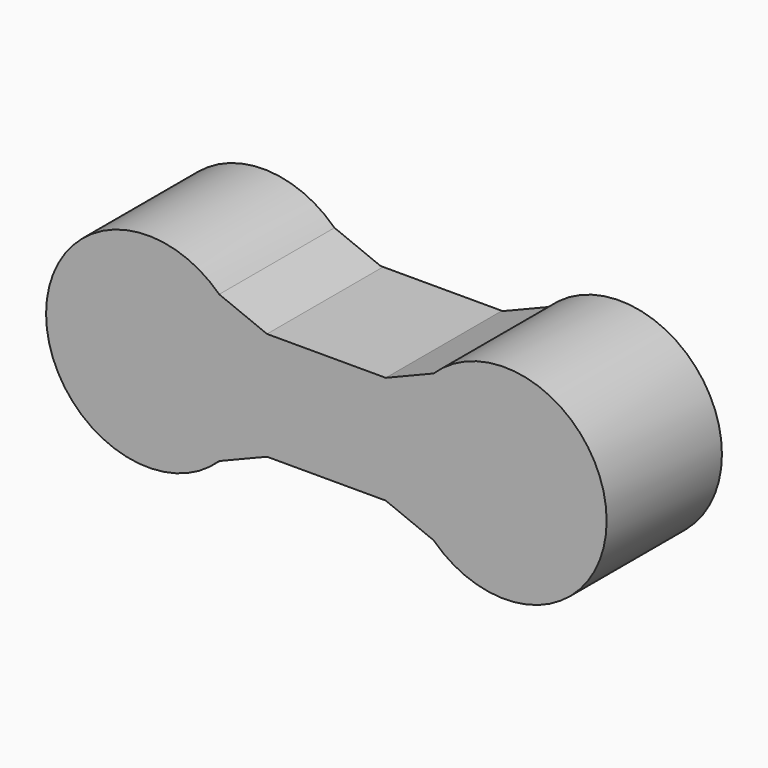
from build123d import *

# Parameters (mm, degrees)
F0_W        = 59.7408041358
F0_H        = 14.4018009305
F1_DEPTH    = 9.66812
F2_R        = 13.6043152125
F3_DEPTH    = 19.19795
F4_T1_DEPTH = 19.19795


# Not quite as in the source:
# - a fillet or chamfer that OpenCascade refuses, or shapes differently, is made with other operations: its cross-section is extruded or revolved along the edge and cut away or added


with BuildPart() as f1:
    # F0 (on Front) → F1 (new body, symmetric)
    with BuildSketch(Plane.XZ):
        Rectangle(F0_W, F0_H)
    extrude(amount=F1_DEPTH, both=True)

    # F2 (on face) → F3 (join)
    with BuildSketch(Plane.XZ.offset(9.66812)):
        with Locations((-23.7363018095, 0)):
            Circle(F2_R)
        with Locations((23.7363018095, 0)):
            Circle(F2_R)
    extrude(amount=-F3_DEPTH)

    # F4: chamfer of 5.08 on 4 edges, made by hand

    # F4_s2 → F4_t1 (join)
    with BuildSketch(Plane.XZ.offset(-9.52983)):
        with BuildLine():
            Line((14.4648728864, 9.8532071559), (7.7209301601, 7.1246894588))
            Line((7.7209301601, 7.1246894588), (7.7209301601, 7.0230894588))
            ThreePointArc((7.7209301601, 7.0230894588), (9.9574717116, 7.0993004653), (12.194013263, 7.0993004653))
            Line((12.194013263, 7.0993004653), (12.2802135971, 7.1471225664))
            ThreePointArc((12.2802135971, 7.1471225664), (13.291854629, 8.5578526047), (14.5355207103, 9.7801904113))
            Line((14.5355207103, 9.7801904113), (14.4648728864, 9.8532071559))
        make_face()
        with BuildLine():
            Line((-14.4648728864, 9.8532071559), (-7.7209301601, 7.1246894588))
            Line((-7.7209301601, 7.1246894588), (-7.7209301601, 7.0230894588))
            ThreePointArc((-7.7209301601, 7.0230894588), (-9.9574717116, 7.0993004653), (-12.194013263, 7.0993004653))
            Line((-12.194013263, 7.0993004653), (-12.2802135971, 7.1471225664))
            ThreePointArc((-12.2802135971, 7.1471225664), (-13.291854629, 8.5578526047), (-14.5355207103, 9.7801904113))
            Line((-14.5355207103, 9.7801904113), (-14.4648728864, 9.8532071559))
        make_face()
        with BuildLine():
            Line((14.4648728864, -9.8532071559), (7.7209301601, -7.1246894588))
            Line((7.7209301601, -7.1246894588), (7.7209301601, -7.0230894588))
            ThreePointArc((7.7209301601, -7.0230894588), (9.9574717116, -7.0993004653), (12.194013263, -7.0993004653))
            Line((12.194013263, -7.0993004653), (12.2802135971, -7.1471225664))
            ThreePointArc((12.2802135971, -7.1471225664), (13.291854629, -8.5578526047), (14.5355207103, -9.7801904113))
            Line((14.5355207103, -9.7801904113), (14.4648728864, -9.8532071559))
        make_face()
        with BuildLine():
            Line((-14.4648728864, -9.8532071559), (-7.7209301601, -7.1246894588))
            Line((-7.7209301601, -7.1246894588), (-7.7209301601, -7.0230894588))
            ThreePointArc((-7.7209301601, -7.0230894588), (-9.9574717116, -7.0993004653), (-12.194013263, -7.0993004653))
            Line((-12.194013263, -7.0993004653), (-12.2802135971, -7.1471225664))
            ThreePointArc((-12.2802135971, -7.1471225664), (-13.291854629, -8.5578526047), (-14.5355207103, -9.7801904113))
            Line((-14.5355207103, -9.7801904113), (-14.4648728864, -9.8532071559))
        make_face()
    extrude(amount=F4_T1_DEPTH)


solid = f1.part
